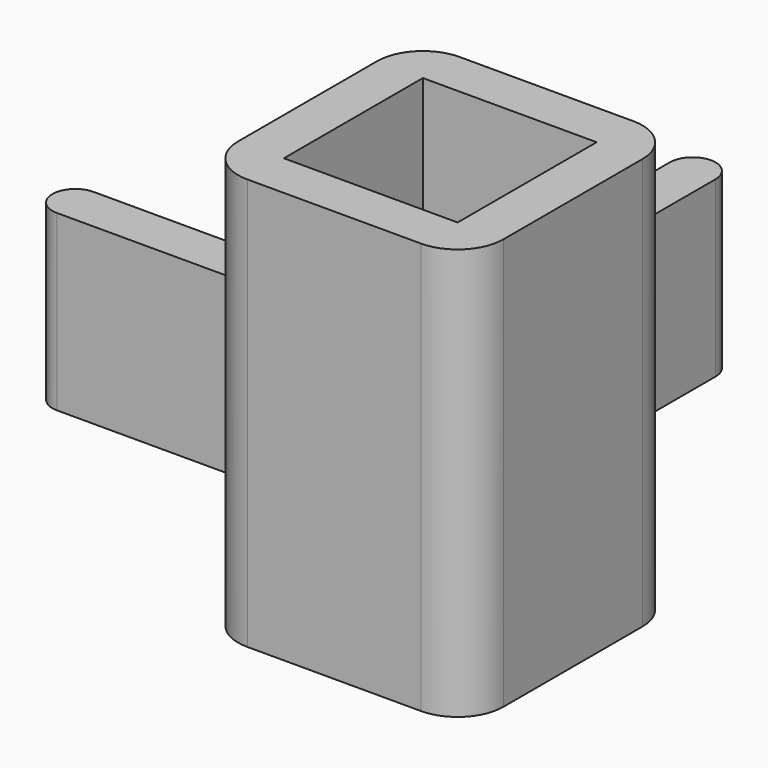
from build123d import *

# Parameters (mm, degrees)
F0_W     = 15.2
F0_H     = 15.2
F0_W_2   = 30
F0_H_2   = 4
F0_W_3   = 4
F0_H_3   = 30
F1_DEPTH = 4
F2_DEPTH = 36
F3_DEPTH = 15.2
F4_R     = 3.99999
F6_R     = 1.99999


# Not quite as in the source:
# - a fillet or chamfer is up to 0.001 mm smaller than in the source, because OpenCascade refuses the exact size
# - a feature of the source that left no trace in its solid (it failed there, or was rolled back) is left out


with BuildPart() as f1:
    # F0 (on Top) → F1 (new body)
    with BuildSketch(Plane.XY):
        Polygon((-4, 15.2), (-4, -4), (19.2, -4), (19.2, 19.2), (0, 19.2), (-4, 19.2), align=None)
        with Locations((7.6, 7.6)):
            Rectangle(F0_W, F0_H, mode=Mode.SUBTRACT)
        with Locations((-19, 17.2)):
            Rectangle(F0_W_2, F0_H_2)
        with Locations((-2, 34.2)):
            Rectangle(F0_W_3, F0_H_3)
        with Locations((7.6, 7.6)):
            Rectangle(F0_W, F0_H)
    extrude(amount=F1_DEPTH)

    # F0 (on Top) → F2 (join)
    with BuildSketch(Plane.XY):
        Polygon((-4, 15.2), (-4, -4), (19.2, -4), (19.2, 19.2), (0, 19.2), (-4, 19.2), align=None)
        with Locations((7.6, 7.6)):
            Rectangle(F0_W, F0_H, mode=Mode.SUBTRACT)
    extrude(amount=F2_DEPTH)

    # F0 (on Top) → F3 (join)
    with BuildSketch(Plane.XY):
        with Locations((-19, 17.2)):
            Rectangle(F0_W_2, F0_H_2)
        with Locations((-2, 34.2)):
            Rectangle(F0_W_3, F0_H_3)
    extrude(amount=F3_DEPTH)

    # F4 (radius 4 in the source; OpenCascade refuses exactly that, so slightly less here)
    f4_edges = [f1.edges().sort_by_distance(p)[0] for p in [
        (-4, -4, 18),
        (19.2, -4, 18),
        (19.2, 19.2, 18),
        (-4, 19.2, 7.6),
        (-4, 19.2, 25.6),
    ]]
    fillet(f4_edges, radius=F4_R)

    # F6 (radius 2 in the source; OpenCascade refuses exactly that, so slightly less here)
    f6_edges = [f1.edges().sort_by_distance(p)[0] for p in [
        (0, 49.2, 7.6),
        (-4, 49.2, 7.6),
        (-34, 19.2, 7.6),
        (-34, 15.2, 7.6),
    ]]
    fillet(f6_edges, radius=F6_R)


solid = f1.part
